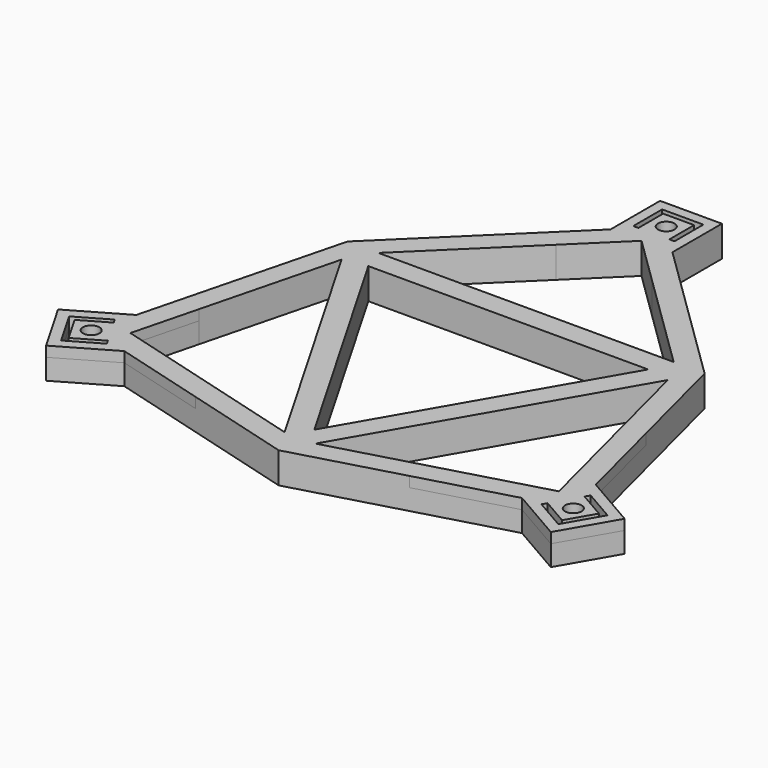
from build123d import *

# Parameters (mm, degrees)
F1_DEPTH  = 10
F2_R      = 4
F3_DEPTH  = 25
F7_DEPTH  = 25
F8_R      = 4
F9_DEPTH  = 5
F10_DEPTH = 5


# Not quite as in the source:
# - after a boolean that leaves OpenCascade's solid faulty, fix() repairs it


with BuildPart() as f1:
    # F0 (on Top) → F1 (new body)
    with BuildSketch(Plane.XY):
        Polygon((0, 0), (86.6025403784, 50), (71.6025403784, 50), (0, 50), align=None)
        Polygon((-86.6025403784, 50), (0, 0), (0, 50), (-71.6025403784, 50), align=None)
        Polygon((0, 120), (15, 120), (15, 150), (-15, 150), (-15, 120), align=None)
        Polygon((10, 125), (0, 125), (-10, 125), (-10, 127.5), (-10, 145), (10, 145), (10, 127.5), align=None, mode=Mode.SUBTRACT)
        with BuildLine():
            Line((71.6025403784, 50), (86.6025403784, 50))
            Line((86.6025403784, 50), (48.027253047, 87.7119317126))
            ThreePointArc((48.027253047, 87.7119317126), (35.9639012974, 93.309151767), (23.2645159855, 97.2561684211))
            Line((23.2645159855, 97.2561684211), (71.6025403784, 50))
        make_face()
        with BuildLine():
            Line((-48.027253047, 87.7119317126), (-86.6025403784, 50))
            Line((-86.6025403784, 50), (-71.6025403784, 50))
            Line((-71.6025403784, 50), (-23.2645159855, 97.2561684211))
            ThreePointArc((-23.2645159855, 97.2561684211), (-35.9639012974, 93.309151767), (-48.027253047, 87.7119317126))
        make_face()
        with BuildLine():
            ThreePointArc((23.2645159855, 97.2561684211), (35.9639012974, 93.309151767), (48.027253047, 87.7119317126))
            Line((48.027253047, 87.7119317126), (15, 120))
            Line((15, 120), (0, 120))
            Line((0, 120), (23.2645159855, 97.2561684211))
        make_face()
        with BuildLine():
            Line((-23.2645159855, 97.2561684211), (0, 120))
            Line((0, 120), (-15, 120))
            Line((-15, 120), (-48.027253047, 87.7119317126))
            ThreePointArc((-48.027253047, 87.7119317126), (-35.9639012974, 93.309151767), (-23.2645159855, 97.2561684211))
        make_face()
        Polygon((-7.5, 127.5), (7.5, 127.5), (0, 135), align=None)
        Polygon((0, 135), (7.5, 127.5), (7.5, 142.5), align=None)
        Polygon((-7.5, 142.5), (-7.5, 127.5), (0, 135), align=None)
        Polygon((0, 135), (7.5, 142.5), (-7.5, 142.5), align=None)
        Polygon((-10, 125), (0, 125), (10, 125), (10, 127.5), (7.5, 127.5), (-7.5, 127.5), (-10, 127.5), align=None)
    extrude(amount=F1_DEPTH)

    # F2 (on face) → F3 (cut)
    with BuildSketch(Plane.XY.offset(10)):
        with Locations((0, 135)):
            Circle(F2_R)
    extrude(amount=-F3_DEPTH, mode=Mode.SUBTRACT)


with BuildPart() as f4_1:
    # F4: instance of F1
    add(f1.part.mirror(Plane(origin=(-43.3012701892, 25, 5), x_dir=(0.8660254038, -0.5, 0), z_dir=(-0.5, -0.8660254038, 0))))


with BuildPart() as f1_1:
    add(f1.part)

    add(f4_1.part)  # F5 merges F4_1
    # F5: F1 across face
    add(f1.part.mirror(Plane(origin=(43.3012701892, 25, 5), x_dir=(0.8660254038, 0.5, 0), z_dir=(0.5, -0.8660254038, 0))))

    # F6 (on face) → F7 (cut)
    with BuildSketch(Plane.XY.offset(10)):
        Polygon((67.8525403784, 39.1746824527), (-67.8525403784, 39.1746824527), (0, -78.3493649054), align=None)
    extrude(amount=-F7_DEPTH, mode=Mode.SUBTRACT)

    # F8 (on face) → F9 (join)
    with BuildSketch(Plane.XY.offset(10)):
        with BuildLine():
            Line((0, 120), (-15, 120))
            Line((-15, 120), (-48.027253047, 87.7119317126))
            ThreePointArc((-48.027253047, 87.7119317126), (-35.9639012974, 93.3091517669), (-23.2645159855, 97.2561684211))
            Line((-23.2645159855, 97.2561684211), (0, 120))
        make_face()
        with BuildLine():
            Line((15, 120), (0, 120))
            Line((0, 120), (23.2645159855, 97.2561684211))
            ThreePointArc((23.2645159855, 97.2561684211), (35.9639012974, 93.3091517669), (48.027253047, 87.7119317126))
            Line((48.027253047, 87.7119317126), (15, 120))
        make_face()
        Polygon((15, 150), (-15, 150), (-15, 120), (0, 120), (15, 120), align=None)
        with Locations((0, 135)):
            Circle(F8_R, mode=Mode.SUBTRACT)
        Polygon((-7.5, 127.5), (-10, 127.5), (-10, 145), (10, 145), (10, 127.5), (7.5, 127.5), (7.5, 142.5), (-7.5, 142.5), align=None, mode=Mode.SUBTRACT)
        Polygon((137.4038105677, -62.0096189432), (111.4230484541, -47.0096189432), (103.9230484541, -60), (96.4230484541, -72.9903810568), (122.4038105677, -87.9903810568), align=None)
        Polygon((119.6586200393, -77.7451905284), (127.1586200393, -64.7548094716), (114.1682389825, -57.2548094716), (115.4182389825, -55.0897459622), (130.5736835487, -63.8397459622), (120.5736835487, -81.1602540378), (105.4182389825, -72.4102540378), (106.6682389825, -70.2451905284), align=None, mode=Mode.SUBTRACT)
        with Locations((116.9134295109, -67.5)):
            Circle(F8_R, mode=Mode.SUBTRACT)
        with BuildLine():
            Line((111.4230484541, -47.0096189432), (99.9743876016, -2.2631446437))
            ThreePointArc((99.9743876016, -2.2631446437), (98.7900464845, -15.5089237407), (95.8585705202, -28.4804223604))
            Line((95.8585705202, -28.4804223604), (103.9230484541, -60))
            Line((103.9230484541, -60), (111.4230484541, -47.0096189432))
        make_face()
        with BuildLine():
            Line((103.9230484541, -60), (72.5940545347, -68.7757460608))
            ThreePointArc((72.5940545347, -68.7757460608), (62.826145187, -77.8002280263), (51.9471345547, -85.448787069))
            Line((51.9471345547, -85.448787069), (96.4230484541, -72.9903810568))
            Line((96.4230484541, -72.9903810568), (103.9230484541, -60))
        make_face()
        Polygon((-103.9230484541, -60), (-111.4230484541, -47.0096189432), (-137.4038105677, -62.0096189432), (-122.4038105677, -87.9903810568), (-96.4230484541, -72.9903810568), align=None)
        Polygon((-120.5736835487, -81.1602540378), (-130.5736835487, -63.8397459622), (-115.4182389825, -55.0897459622), (-114.1682389825, -57.2548094716), (-127.1586200393, -64.7548094716), (-119.6586200393, -77.7451905284), (-106.6682389825, -70.2451905284), (-105.4182389825, -72.4102540378), align=None, mode=Mode.SUBTRACT)
        with Locations((-116.9134295109, -67.5)):
            Circle(F8_R, mode=Mode.SUBTRACT)
        with BuildLine():
            ThreePointArc((-95.8585705202, -28.4804223604), (-98.7900464845, -15.5089237407), (-99.9743876016, -2.2631446437))
            Line((-99.9743876016, -2.2631446437), (-111.4230484541, -47.0096189432))
            Line((-111.4230484541, -47.0096189432), (-103.9230484541, -60))
            Line((-103.9230484541, -60), (-95.8585705202, -28.4804223604))
        make_face()
        with BuildLine():
            Line((-72.5940545347, -68.7757460608), (-103.9230484541, -60))
            Line((-103.9230484541, -60), (-96.4230484541, -72.9903810568))
            Line((-96.4230484541, -72.9903810568), (-51.9471345547, -85.448787069))
            ThreePointArc((-51.9471345547, -85.448787069), (-62.826145187, -77.8002280263), (-72.5940545347, -68.7757460608))
        make_face()
    extrude(amount=F9_DEPTH)

    # F10 (add): a face of the model
    f10_faces = [f1_1.faces().sort_by_distance(p)[0] for p in [
        (25.2159598464, -90.0197712228, 10),
    ]]
    extrude(f10_faces, amount=F10_DEPTH)

    add(f1_1.part.fix(), mode=Mode.REPLACE)


solid = f1_1.part
